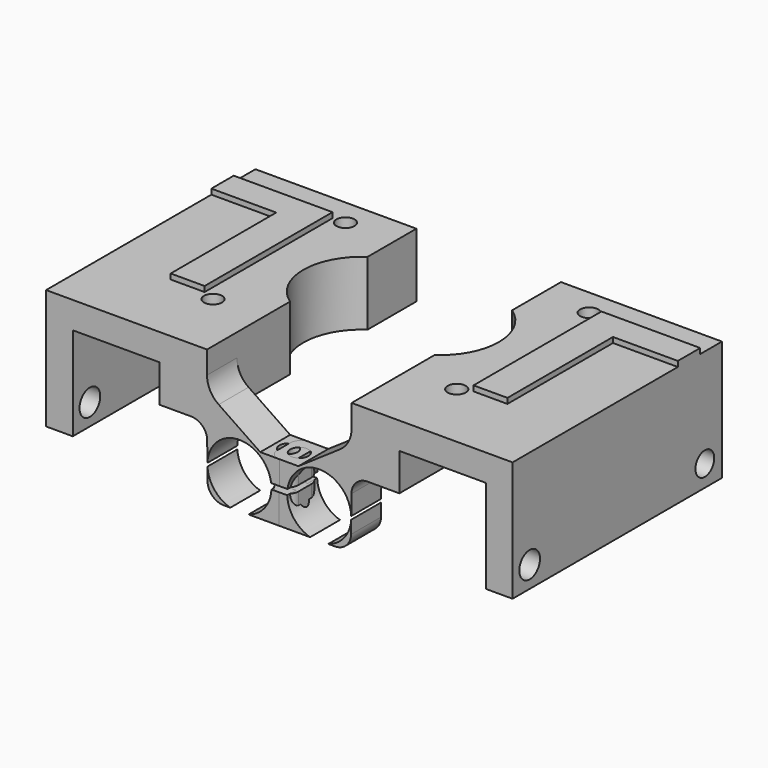
from build123d import *

# Parameters (mm, degrees)
F1_DEPTH      = 7
F2_DEPTH      = 42
F3_R          = 1.7
F3_R_2        = 11
F4_DEPTH      = 12.001
F5_R          = 6
F6_DEPTH      = 10
F7_DEPTH      = 12.001
F8_R          = 1.4
F9_DEPTH      = 10.9920075553
F8_R_2        = 1.7
F10_DEPTH     = 4.4358210087
F11_R         = 5
F12_R         = 3
F13_R         = 3
F14_R         = 2
F15_R         = 2.2
F15_R_2       = 2.4255023423
F16_DEPTH     = 6
F17_TEXT_SIZE = 41.9437823343
F18_DEPTH     = 1


# Not quite as in the source:
# - a feature names something its author has since deleted; it is built from what else it names
# - Text() gives the source's letters only with a copy of the font that has no kerning and outlines rounded to 1/6400 em; it was checked with that copy


with BuildPart() as f1:
    # F0 (on Front) → F1 (new body)
    with BuildSketch(Plane.XZ):
        Polygon((-18.6721007523, 29.8099789735), (-18.6721007523, 7.3259699669), (-13.6721007523, 7.3259699669), (-13.6721007523, 24.8099789735), (2.5278992477, 24.8099789735), (2.5278992477, 17.8099789735), (11.4637966118, 17.8099789735), (11.4637966118, 22.9406704692), (11.4637966118, 29.8099789735), align=None)
        Polygon((21.4301751077, 16.1394868046), (11.4637966118, 22.9406704692), (11.4637966118, 17.8099789735), (11.5940201178, 5.1484792493), (27.0186601057, 5.1484792493), (27.0186601057, 10.6682249423), (19.6860510706, 10.6682249423), (19.6860510706, 11.7046658959), (26.9896428882, 11.7046658959), (26.9896428882, 16.1394868046), align=None)
    extrude(amount=F1_DEPTH)

    # F0 (on Front) → F2 (join)
    with BuildSketch(Plane.XZ):
        Polygon((-18.6721007523, 29.8099789735), (-18.6721007523, 7.3259699669), (-13.6721007523, 7.3259699669), (-13.6721007523, 24.8099789735), (2.5278992477, 24.8099789735), (2.5278992477, 17.8099789735), (11.4637966118, 17.8099789735), (11.4637966118, 22.9406704692), (11.4637966118, 29.8099789735), align=None)
    extrude(amount=-F2_DEPTH)

    # F3 (on face) → F4 (cut, through all)
    with BuildSketch(Plane(origin=(0, 0, 17.8099789735), x_dir=(1, 0, 0), z_dir=(0, 0, -1))):
        with Locations((2.1850741468, -6)):
            Circle(F3_R)
        with Locations((2.1850741468, -37)):
            Circle(F3_R)
        with Locations((17.6850741468, -21.5)):
            Circle(F3_R_2)
    extrude(amount=-F4_DEPTH, mode=Mode.SUBTRACT)

    # F5 (on face) → F6 (cut)
    with BuildSketch(Plane.XZ.offset(7)):
        with Locations((17.5278992477, 10.8989789735)):
            Circle(F5_R)
    extrude(amount=-F6_DEPTH, mode=Mode.SUBTRACT)

    # F3 (on face) → F7 (cut, through all)
    with BuildSketch(Plane(origin=(0, 0, 17.8099789735), x_dir=(1, 0, 0), z_dir=(0, 0, -1))):
        with Locations((2.1850741468, -6)):
            Circle(F3_R)
        with Locations((2.1850741468, -37)):
            Circle(F3_R)
        with Locations((17.6850741468, -21.5)):
            Circle(F3_R_2)
    extrude(amount=-F7_DEPTH, mode=Mode.SUBTRACT)

    # F8 (on face) → F9 (cut, through all)
    with BuildSketch(Plane.XY.offset(16.1394868046)):
        with Locations((23.9896428882, -3.5767070949)):
            Circle(F8_R)
    extrude(amount=-F9_DEPTH, mode=Mode.SUBTRACT)

    # F8 (on face) → F10 (cut, through all)
    with BuildSketch(Plane.XY.offset(16.1394868046)):
        with Locations((23.9896428882, -3.5767070949)):
            Circle(F8_R_2)
        with Locations((23.9896428882, -3.5767070949)):
            Circle(F8_R, mode=Mode.SUBTRACT)
    extrude(amount=-F10_DEPTH, mode=Mode.SUBTRACT)

    # F11
    f11_edges = [f1.edges().sort_by_distance(p)[0] for p in [
        (11.463797, -3.5, 22.94067),
    ]]
    fillet(f11_edges, radius=F11_R)

    # F12
    f12_edges = [f1.edges().sort_by_distance(p)[0] for p in [
        (11.463797, -3.5, 17.809979),
    ]]
    fillet(f12_edges, radius=F12_R)

    # F13
    f13_edges = [f1.edges().sort_by_distance(p)[0] for p in [
        (11.59402, -3.5, 5.148479),
    ]]
    fillet(f13_edges, radius=F13_R)

    # F14
    f14_edges = [f1.edges().sort_by_distance(p)[0] for p in [
        (26.989643, -7, 13.922076),
        (27.01866, -7, 7.908352),
        (26.989643, 0, 13.922076),
        (27.01866, 0, 7.908352),
    ]]
    fillet(f14_edges, radius=F14_R)

    # F15 (on face) → F16 (cut)
    with BuildSketch(Plane(origin=(-18.6721007523, 0, 0), x_dir=(0, -1, 0), z_dir=(-1, 0, 0))):
        with Locations((-38, 11.3259699669)):
            Circle(F15_R)
        with Locations((3, 11.3259699669)):
            Circle(F15_R_2)
    extrude(amount=-F16_DEPTH, mode=Mode.SUBTRACT)

    # F17 (on face) → F18 (join)
    with BuildSketch(Plane.XY.offset(29.8099789735)):
        with Locations(Location((3.5908724648, 36.9253193088), (0, 0, 180))):
            Text('L', F17_TEXT_SIZE, font='Open Sans', font_style=FontStyle.BOLD, text_align=(TextAlign.LEFT, TextAlign.BOTTOM))
    extrude(amount=F18_DEPTH)


with BuildPart() as f19_1:
    # F19: instance of F1
    add(f1.part.mirror(Plane.YZ))


with BuildPart() as f19_1_1:
    # F20: moved
    add(f19_1.part.moved(Location((50, 0, 0))))


solid = Compound([f1.part, f19_1_1.part])
